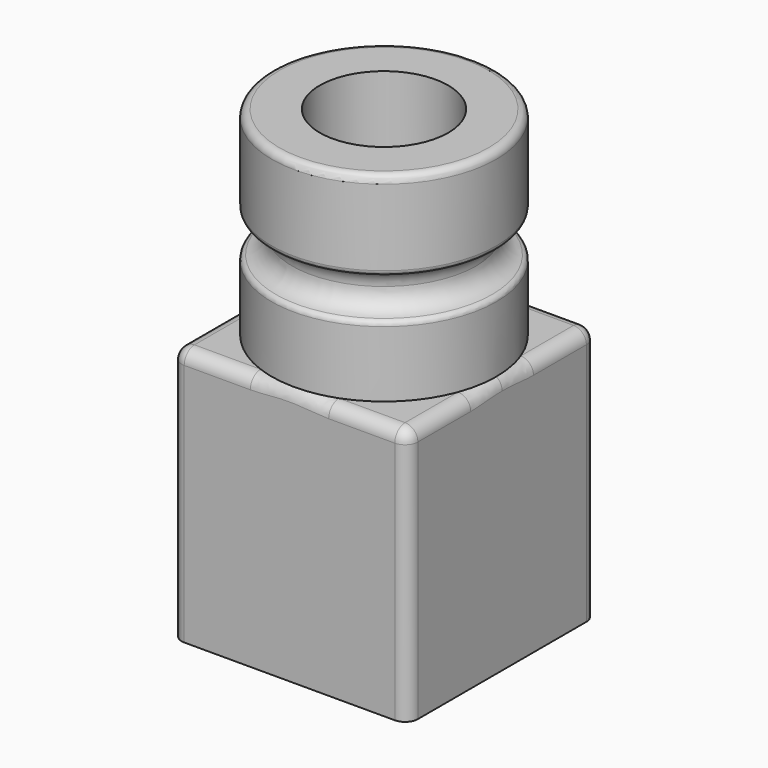
from build123d import *

# Parameters (mm, degrees)
F0_R      = 8.75
F1_DEPTH  = 15.5
F3_START  = -6.9
F2_R      = 12.7162229671
F2_R_2    = 7.15
F3_DEPTH  = 3.1
F4_W      = 18.4
F4_H      = 18.4
F5_DEPTH  = 20
F6_W      = 15.2
F6_H      = 15.2
F7_DEPTH  = 18
F8_R      = 0.6
F9_R      = 1.54999
F10_R     = 1
F11_R     = 5
F12_DEPTH = 25
F13_R     = 2
F14_R     = 1
F15_R     = 0.4


# Not quite as in the source:
# - a fillet or chamfer is up to 0.001 mm smaller than in the source, because OpenCascade refuses the exact size


with BuildPart() as f1:
    # F0 (on Top) → F1 (new body)
    with BuildSketch(Plane.XY):
        Circle(F0_R)
    extrude(amount=F1_DEPTH)

    # F2 (on face) → F3 (cut)
    with BuildSketch(Plane.XY.offset(15.5).offset(F3_START)):
        Circle(F2_R)
        Circle(F2_R_2, mode=Mode.SUBTRACT)
    extrude(amount=-F3_DEPTH, mode=Mode.SUBTRACT)

    # F4 (on face) → F5 (join)
    with BuildSketch(Plane(origin=(0, 0, 0), x_dir=(1, 0, 0), z_dir=(0, 0, -1))):
        Rectangle(F4_W, F4_H)
    extrude(amount=F5_DEPTH)

    # F6 (on face) → F7 (cut)
    with BuildSketch(Plane(origin=(0, 0, -20), x_dir=(1, 0, 0), z_dir=(0, 0, -1))):
        Rectangle(F6_W, F6_H)
    extrude(amount=-F7_DEPTH, mode=Mode.SUBTRACT)

    # F8
    f8_edges = [f1.edges().sort_by_distance(p)[0] for p in [
        (-8.75, 0, 15.5),
    ]]
    fillet(f8_edges, radius=F8_R)

    # F9 (radius 1.55 in the source; OpenCascade refuses exactly that, so slightly less here)
    f9_edges = [f1.edges().sort_by_distance(p)[0] for p in [
        (-7.15, 0, 5.5),
        (-7.15, 0, 8.6),
    ]]
    fillet(f9_edges, radius=F9_R)

    # F10
    f10_edges = [f1.edges().sort_by_distance(p)[0] for p in [
        (9.2, -9.2, -10),
        (9.2, 9.2, -10),
        (-9.2, 9.2, -10),
        (-9.2, -9.2, -10),
    ]]
    fillet(f10_edges, radius=F10_R)

    # F11 (on face) → F12 (cut)
    with BuildSketch(Plane.XY.offset(15.5)):
        Circle(F11_R)
    extrude(amount=-F12_DEPTH, mode=Mode.SUBTRACT)

    # F13
    f13_edges = [f1.edges().sort_by_distance(p)[0] for p in [
        (-5, 0, -2),
    ]]
    fillet(f13_edges, radius=F13_R)

    # F14
    f14_edges = [f1.edges().sort_by_distance(p)[0] for p in [
        (0, -9.2, 0),
    ]]
    fillet(f14_edges, radius=F14_R)

    # F15
    f15_edges = [f1.edges().sort_by_distance(p)[0] for p in [
        (-8.75, 0, 8.6),
        (-8.75, 0, 5.5),
    ]]
    fillet(f15_edges, radius=F15_R)


solid = f1.part
